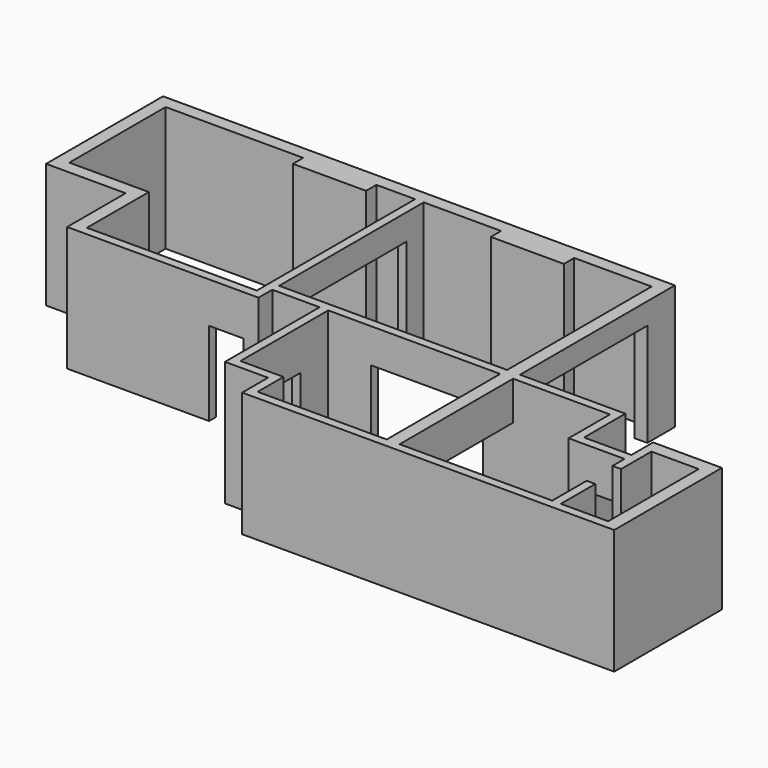
from build123d import *

# Parameters (mm, degrees)
F1_DEPTH  = 2900
F2_W      = 300
F2_H      = 500
F3_DEPTH  = 3000
F4_W      = 200
F4_H      = 600
F5_DEPTH  = 3500
F6_W      = 200
F6_H      = 950
F7_DEPTH  = 1000
F8_W      = 200
F8_H      = 950
F9_DEPTH  = 1000
F10_W     = 200
F10_H     = 800
F11_DEPTH = 3000
F12_W     = 300
F12_H     = 900
F13_DEPTH = 2580
F14_W     = 200
F14_H     = 950
F15_DEPTH = 830


# Not quite as in the source:
# - a feature names something its author has since deleted; it is built from what else it names


with BuildPart() as f1:
    # F0 (on Top) → F1 (new body)
    with BuildSketch(Plane.XY):
        Polygon((3635.0218463784, 3800), (-8264.9781536216, 3800), (-8264.9781536216, 400), (-6414.9781536216, 400), (-6414.9781536216, -1300), (-3114.9781536216, -1300), (-3114.9781536216, -1100), (-6114.9781536216, -1100), (-6114.9781536216, 700), (-7964.9781536216, 700), (-7964.9781536216, 3500), (-4764.9781536216, 3500), (-4764.9781536216, 3200), (-3064.9781536216, 3200), (-3064.9781536216, 3500), (-2164.9781536216, 3500), (-2164.9781536216, 3000), (-1964.9781536216, 3000), (-1964.9781536216, 3500), (-164.9781536216, 3500), (-164.9781536216, 3200), (1535.0218463784, 3200), (1535.0218463784, 3500), (3335.0218463784, 3500), (3335.0218463784, 3000), (3635.0218463784, 3000), align=None)
    extrude(amount=F1_DEPTH)



with BuildPart() as f1b:
    # F0 (on Top) → F1, piece 2 (new body)
    with BuildSketch(Plane.XY):
        Polygon((-2164.9781536216, 0), (-2164.9781536216, -1100), (-2314.9781536216, -1100), (-2314.9781536216, -1300), (-1964.9781536216, -1300), (-1964.9781536216, -900), (-864.9781536216, -900), (-864.9781536216, -1700), (-664.9781536216, -1700), (-664.9781536216, -900), (335.0218463784, -900), (335.0218463784, -700), (-1964.9781536216, -700), (-1964.9781536216, 0), align=None)
    extrude(amount=F1_DEPTH)


with BuildPart() as f1c:
    # F0 (on Top) → F1, piece 3 (new body)
    with BuildSketch(Plane.XY):
        Polygon((3335.0218463784, -700), (2935.0218463784, -700), (2935.0218463784, -900), (5885.0218463784, -900), (5885.0218463784, -2100), (6235.0218463784, -2100), (6235.0218463784, -1900), (6085.0218463784, -1900), (6085.0218463784, -700), (3635.0218463784, -700), (3635.0218463784, 0), (3335.0218463784, 0), align=None)
    extrude(amount=F1_DEPTH)


with BuildPart() as f1d:
    # F0 (on Top) → F1, piece 4 (new body)
    with BuildSketch(Plane.XY):
        Polygon((7185.0218463784, -4200), (3635.0218463784, -4200), (3635.0218463784, -3400), (3335.0218463784, -3400), (3335.0218463784, -4200), (335.0218463784, -4200), (335.0218463784, -3450), (-664.9781536216, -3450), (-664.9781536216, -2500), (-864.9781536216, -2500), (-864.9781536216, -3650), (135.0218463784, -3650), (135.0218463784, -4400), (8785.0218463784, -4400), (8785.0218463784, -1268.9918279648), (7185.0218463784, -1268.9918279648), (7185.0218463784, -1900), (7035.0218463784, -1900), (7035.0218463784, -2100), (7185.0218463784, -2100), (7185.0218463784, -2450), (7385.0218463784, -2450), (7385.0218463784, -1568.9918279648), (8485.0218463784, -1568.9918279648), (8485.0218463784, -4200), (7385.0218463784, -4200), (7385.0218463784, -3200), (7185.0218463784, -3200), align=None)
    extrude(amount=F1_DEPTH)


with BuildPart() as f1_1:
    add(f1.part)

    add(f1c.part)  # F3 merges F1c
    # F2 (on face) → F3 (join)
    with BuildSketch(Plane.XZ.offset(-3000)):
        with Locations((3485.0218463784, 2650)):
            Rectangle(F2_W, F2_H)
    extrude(amount=F3_DEPTH)


    add(f1b.part)  # F5 merges F1b
    # F4 (on face) → F5 (join)
    with BuildSketch(Plane.XZ.offset(-3000)):
        with Locations((-2064.9781536216, 2600)):
            Rectangle(F4_W, F4_H)
    extrude(amount=F5_DEPTH)


    add(f1d.part)  # F7 merges F1d
    # F6 (on face) → F7 (join)
    with BuildSketch(Plane.XZ.offset(1700)):
        with Locations((-764.9781536216, 2425)):
            Rectangle(F6_W, F6_H)
    extrude(amount=F7_DEPTH)

    # F8 (on face) → F9 (join)
    with BuildSketch(Plane.YZ.offset(-3114.9781536216)):
        with Locations((-1200, 2425)):
            Rectangle(F8_W, F8_H)
    extrude(amount=F9_DEPTH)

    # F10 (on face) → F11 (join)
    with BuildSketch(Plane.YZ.offset(335.0218463784)):
        with Locations((-800, 2500)):
            Rectangle(F10_W, F10_H)
    extrude(amount=F11_DEPTH)

    # F12 (on face) → F13 (join)
    with BuildSketch(Plane(origin=(0, -3400, 0), x_dir=(-1, 0, 0), z_dir=(0, 1, 0))):
        with Locations((-3485.0218463784, 2450)):
            Rectangle(F12_W, F12_H)
    extrude(amount=F13_DEPTH)

    # F14 (on face) → F15 (join)
    with BuildSketch(Plane.YZ.offset(6235.0218463784)):
        with Locations((-2000, 2425)):
            Rectangle(F14_W, F14_H)
    extrude(amount=F15_DEPTH)


solid = f1_1.part
